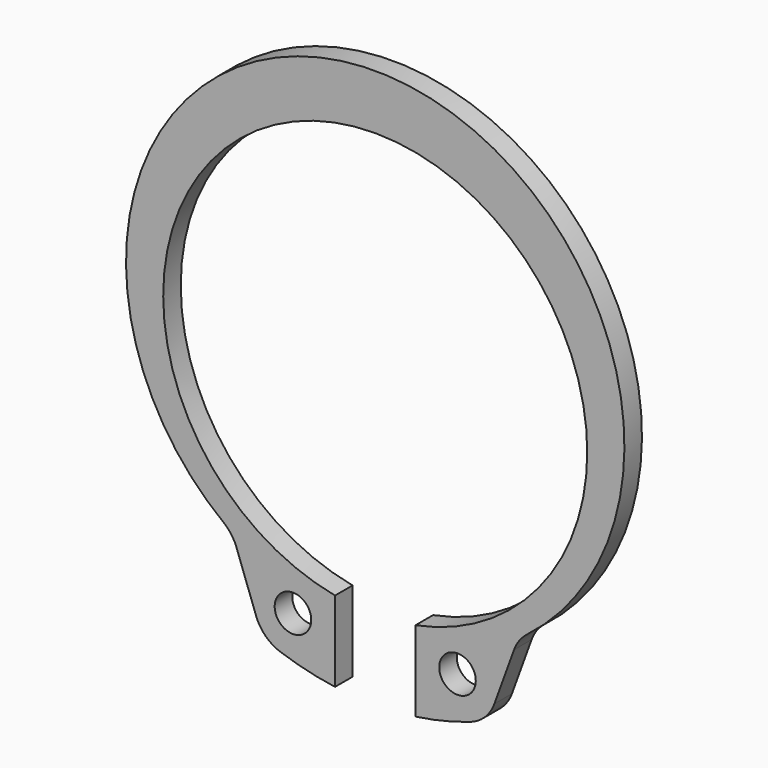
from build123d import *

# Parameters (mm, degrees)
F0_R     = 1
F1_DEPTH = 1.2
F2_R     = 2.15


# Not quite as in the source:
# - a feature names something its author has since deleted; it is built from what else it names


with BuildPart() as f1:
    # F0 (on Front) → F1 (new body)
    with BuildSketch(Plane.XZ):
        with BuildLine():
            ThreePointArc((-2.2, -11.3894688199), (0, 11.6), (2.2, -11.3894688199))
            Line((2.2, -11.3894688199), (2.2, -12.4894688199))
            ThreePointArc((2.2, -12.4894688199), (5.1370226671, -11.6633518005), (7.8168023095, -10.2048071338))
            ThreePointArc((7.8168023095, -10.2048071338), (0, 14.6), (-7.8168023095, -10.2048071338))
            ThreePointArc((-7.8168023095, -10.2048071338), (-5.1370226671, -11.6633518005), (-2.2, -12.4894688199))
            Line((-2.2, -12.4894688199), (-2.2, -11.3894688199))
        make_face()
        with BuildLine():
            ThreePointArc((7.8168023095, -10.2048071338), (5.1370226671, -11.6633518005), (2.2, -12.4894688199))
            Line((2.2, -12.4894688199), (2.2, -15.7894688199))
            ThreePointArc((2.2, -15.7894688199), (4.2270149149, -15.3713913009), (6.1827847392, -14.6942335113))
            Line((6.1827847392, -14.6942335113), (7.8168023095, -10.2048071338))
        make_face()
        with Locations((4.5011299048, -12.9922397434)):
            Circle(F0_R, mode=Mode.SUBTRACT)
        with BuildLine():
            Line((-2.2, -15.7894688199), (-2.2, -12.4894688199))
            ThreePointArc((-2.2, -12.4894688199), (-5.1370226671, -11.6633518005), (-7.8168023095, -10.2048071338))
            Line((-7.8168023095, -10.2048071338), (-6.1827847392, -14.6942335113))
            ThreePointArc((-6.1827847392, -14.6942335113), (-4.2270149149, -15.3713913009), (-2.2, -15.7894688199))
        make_face()
        with Locations((-4.5011299048, -12.9922397434)):
            Circle(F0_R, mode=Mode.SUBTRACT)
    extrude(amount=F1_DEPTH)

    # F2
    f2_edges = [f1.edges().sort_by_distance(p)[0] for p in [
        (6.182785, -0.6, -14.694234),
        (-6.182785, -0.6, -14.694234),
        (-7.816802, -0.6, -10.204807),
        (7.816802, -0.6, -10.204807),
    ]]
    fillet(f2_edges, radius=F2_R)


solid = f1.part
